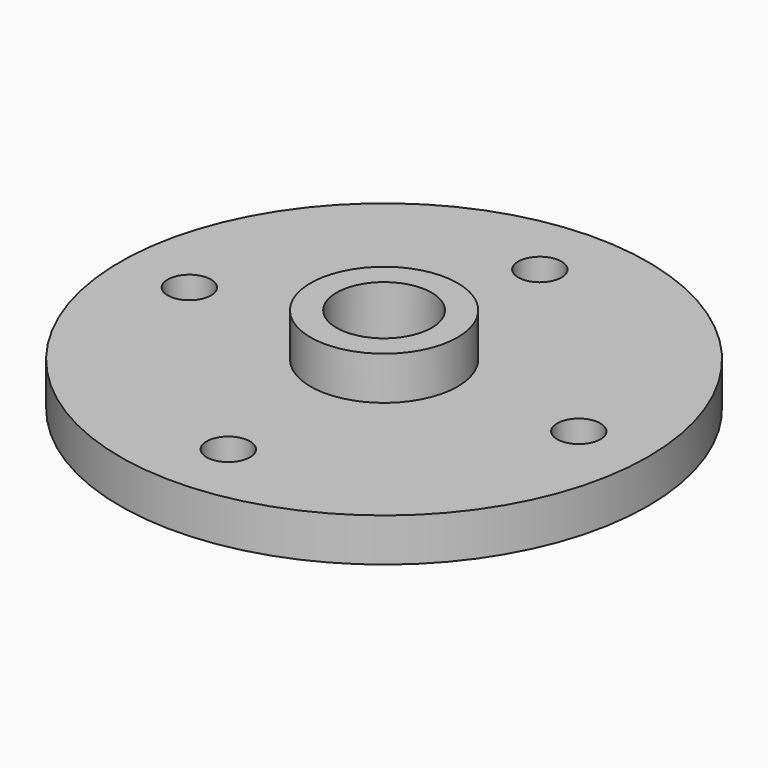
from build123d import *

# Parameters (mm, degrees)
F0_R     = 25.5
F0_R_2   = 8.5
F1_DEPTH = 5
F0_R_3   = 5.5
F2_DEPTH = 10
F3_D     = 5
F0_R_4   = 30.5
F4_DEPTH = 5


# Not quite as in the source:
# - a feature names something its author has since deleted; it is built from what else it names


with BuildPart() as f1:
    # F0 (on Top) → F1 (new body)
    with BuildSketch(Plane.XY):
        Circle(F0_R)
        Circle(F0_R_2, mode=Mode.SUBTRACT)
    extrude(amount=F1_DEPTH)

    # F0 (on Top) → F2 (join)
    with BuildSketch(Plane.XY):
        Circle(F0_R_2)
        Circle(F0_R_3, mode=Mode.SUBTRACT)
    extrude(amount=F2_DEPTH)

    # F3 (through all)
    with Locations(Plane(origin=(0, 0, 0), x_dir=(1, 0, 0), z_dir=(0, 0, -1))):
        with Locations((-22.5, 0), (0, -22.5), (22.5, 0), (0, 22.5)):
            Hole(F3_D / 2)

    # F0 (on Top) → F4 (join, through all)
    with BuildSketch(Plane.XY):
        Circle(F0_R_4)
        Circle(F0_R, mode=Mode.SUBTRACT)
    extrude(amount=F4_DEPTH)


solid = f1.part
